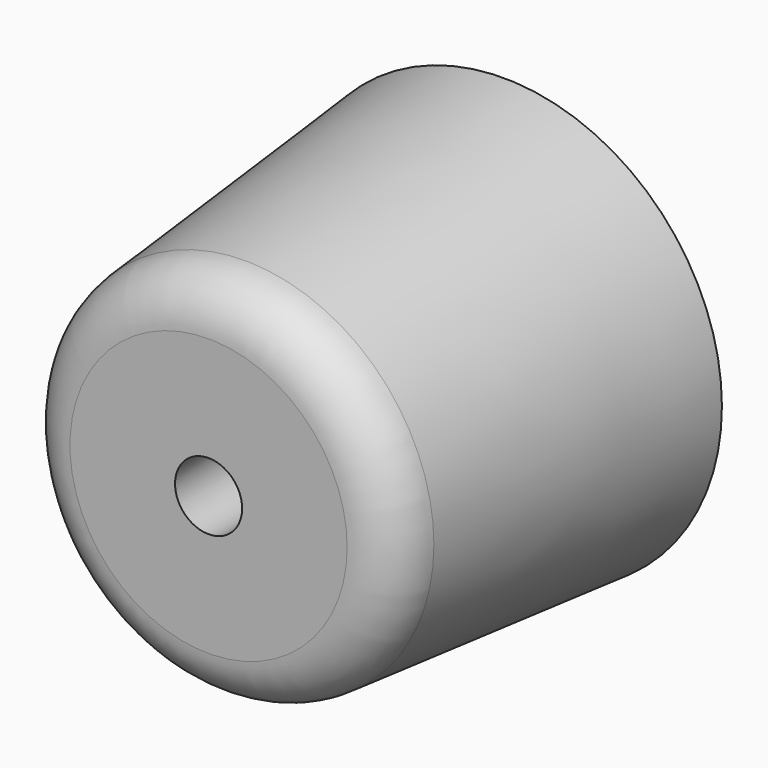
from build123d import *

# Parameters (mm, degrees)
F0_R     = 13
F2_R     = 11
F4_R     = 3
F5_R     = 2
F6_DEPTH = 22.001


with BuildPart() as f3:
    # F0 (on Front) → F3 section 0
    with BuildSketch(Plane.XZ):
        Circle(F0_R)
    # F2 (on offset) → F3 section 1
    with BuildSketch(Plane.XZ.offset(22)):
        Circle(F2_R)
    loft()

    # F4
    f4_edges = [f3.edges().sort_by_distance(p)[0] for p in [
        (-11, -22, 0),
    ]]
    fillet(f4_edges, radius=F4_R)

    # F5 (on Front) → F6 (cut, through all)
    with BuildSketch(Plane.XZ):
        Circle(F5_R)
    extrude(amount=F6_DEPTH, mode=Mode.SUBTRACT)


solid = f3.part
